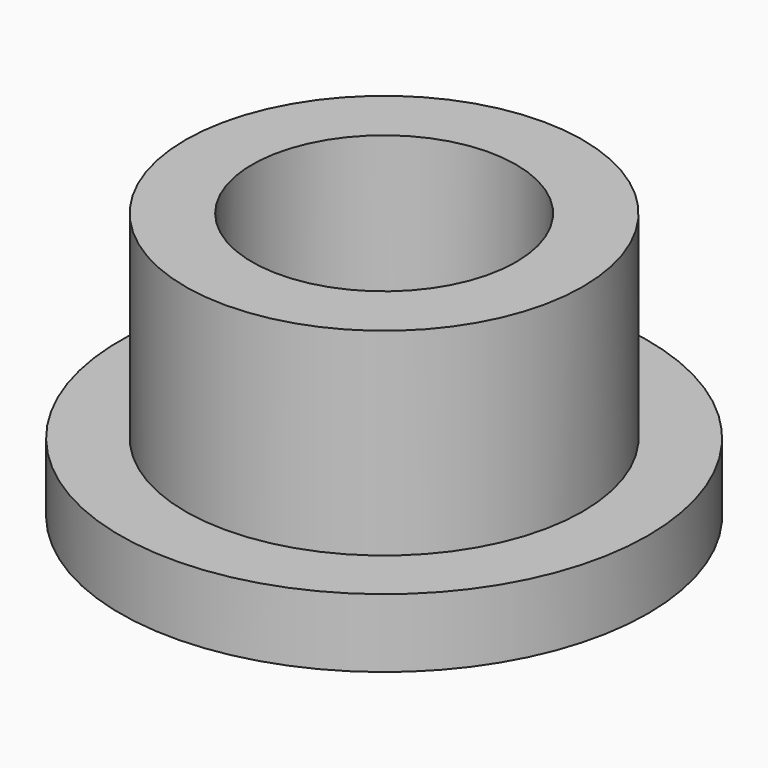
from build123d import *

# Parameters (mm, degrees)
F0_R     = 4.78
F0_R_2   = 3.175
F1_DEPTH = 6.33
F2_DEPTH = 6.41
F0_R_3   = 6.35
F3_DEPTH = 1.65


with BuildPart() as f1:
    # F0 (on Top) → F1 (new body)
    with BuildSketch(Plane.XY):
        Circle(F0_R)
        Circle(F0_R_2, mode=Mode.SUBTRACT)
    extrude(amount=F1_DEPTH)


with BuildPart() as f2:
    # F0 (on Top) → F2 (new body)
    with BuildSketch(Plane.XY):
        Circle(F0_R)
        Circle(F0_R_2, mode=Mode.SUBTRACT)
    extrude(amount=F2_DEPTH)

    # F0 (on Top) → F3 (join)
    with BuildSketch(Plane.XY):
        Circle(F0_R_3)
        Circle(F0_R, mode=Mode.SUBTRACT)
    extrude(amount=F3_DEPTH)


solid = Compound([f1.part, f2.part])
